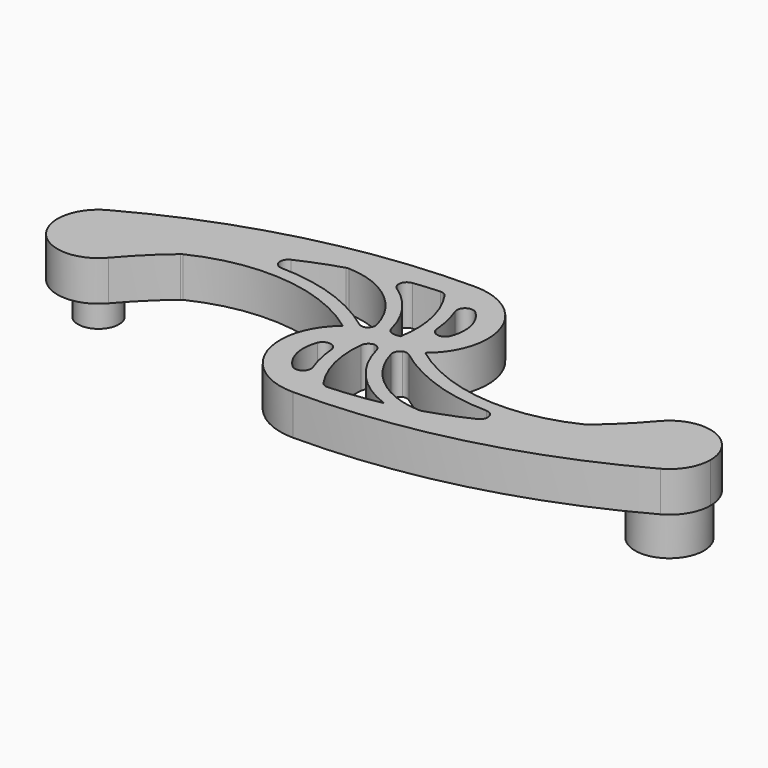
from build123d import *

# Parameters (mm, degrees)
F0_R            = 3.175
F0_R_2          = 5.334
F0_R_3          = 3.2385
F1_DEPTH        = 6.223
F2_DEPTH        = 5.08
F3_DEPTH        = 6.477
F4_DEPTH        = 6.223
F4_COPIES_COUNT = 2
F6_T1_DEPTH     = 6.223


# Not quite as in the source:
# - a fillet or chamfer that OpenCascade refuses, or shapes differently, is made with other operations: its cross-section is extruded or revolved along the edge and cut away or added
# - a pattern or mirror of a feature is missing from the dataset's text; its kind, count and spacing are read off the source's solid
# - a feature names something its author has since deleted; it is built from what else it names


with BuildPart() as f1:
    # F0 (on Top) → F1 (new body)
    with BuildSketch(Plane.XY):
        with BuildLine():
            ThreePointArc((-39.383509083, -4.1130659459), (-38.2614038875, -2.1911061906), (-37.8714, 0))
            ThreePointArc((-37.8714, 0), (-40.9830590014, 5.4622017152), (-47.268454355, 5.5711722068))
            ThreePointArc((-47.268454355, 5.5711722068), (-49.1456147646, -4.0093152723), (-39.383509083, -4.1130659459))
        make_face()
        with Locations((-44.2214, 0)):
            Circle(F0_R, mode=Mode.SUBTRACT)
        with BuildLine():
            ThreePointArc((-47.268454355, 5.5711722068), (-40.9830590014, 5.4622017152), (-37.8714, 0))
            ThreePointArc((-37.8714, 0), (-38.2614038875, -2.1911061906), (-39.383509083, -4.1130659459))
            ThreePointArc((-39.383509083, -4.1130659459), (-36.3513275231, -0.8434709111), (-33.0486454257, 2.1526378433))
            ThreePointArc((-33.0486454257, 2.1526378433), (-30.2955035901, 4.2889551927), (-27.404684246, 6.2349267505))
            ThreePointArc((-27.404684246, 6.2349267505), (-21.4521533969, 9.4356034701), (-15.1329284561, 11.8323410696))
            ThreePointArc((-15.1329284561, 11.8323410696), (-12.7951555369, 12.4884323965), (-10.4291525282, 13.0340218145))
            ThreePointArc((-10.4291525282, 13.0340218145), (-6.1458763765, 13.7303526951), (-1.8192889749, 14.0649759791))
            ThreePointArc((-1.8192889749, 14.0649759791), (-0.9097854022, 14.0889933747), (0, 14.097))
            ThreePointArc((0, 14.097), (0.3233426245, 14.0885072181), (0.6457935928, 14.0630522923))
            ThreePointArc((0.6457935928, 14.0630522923), (6.0043722729, 9.3111643906), (3.2449318821, 2.7020575802))
            ThreePointArc((3.2449318821, 2.7020575802), (2.1979242887, 2.1834953883), (1.0718312901, 1.8719729878))
            ThreePointArc((1.0718312901, 1.8719729878), (0.5379714762, 1.801538222), (0, 1.778))
            ThreePointArc((0, 1.778), (-0.4196313816, 1.7689334209), (-0.8384795567, 1.7417506054))
            ThreePointArc((-0.8384795567, 1.7417506054), (-1.8462351917, 1.6009671655), (-2.8337391369, 1.3555545438))
            ThreePointArc((-2.8337391369, 1.3555545438), (-3.5575469364, 1.1032300615), (-4.2592096932, 0.7946287805))
            ThreePointArc((-4.2592096932, 0.7946287805), (-5.2044321405, 0.2664518736), (-6.0850110833, -0.3636251419))
            ThreePointArc((-6.0850110833, -0.3636251419), (-9.1644672904, -11.1629425329), (0, -17.653))
            ThreePointArc((0, -17.653), (24.3940430225, -14.5847588813), (47.268454355, -5.5711722068))
            ThreePointArc((47.268454355, -5.5711722068), (39.2971852354, -4.0093152723), (39.383509083, 4.1130659459))
            ThreePointArc((39.383509083, 4.1130659459), (21.6948570487, -9.3241427599), (0, -14.097))
            ThreePointArc((0, -14.097), (-6.1595, -7.9375), (0, -1.778))
            ThreePointArc((0, -1.778), (9.7155, 7.9375), (0, 17.653))
            ThreePointArc((0, 17.653), (-24.3940430225, 14.5847588813), (-47.268454355, 5.5711722068))
        make_face()
        with BuildLine():
            ThreePointArc((50.5714, 0), (46.4125061906, 5.9599961125), (39.383509083, 4.1130659459))
            ThreePointArc((39.383509083, 4.1130659459), (39.2971852354, -4.0093152723), (47.268454355, -5.5711722068))
            ThreePointArc((47.268454355, -5.5711722068), (49.6836017152, -3.2383409986), (50.5714, 0))
        make_face()
        with Locations((44.2214, 0)):
            Circle(F0_R_2, mode=Mode.SUBTRACT)
        with Locations((-44.2214, 0)):
            Circle(F0_R)
        with Locations((44.2214, 0)):
            Circle(F0_R_2)
        with Locations((44.2214, 0)):
            Circle(F0_R_3, mode=Mode.SUBTRACT)
        with Locations((44.2214, 0)):
            Circle(F0_R_3)
    extrude(amount=F1_DEPTH)

    # F0 (on Top) → F2 (join)
    with BuildSketch(Plane.XY):
        with Locations((-44.2214, 0)):
            Circle(F0_R)
    extrude(amount=-F2_DEPTH)

    # F0 (on Top) → F3 (join)
    with BuildSketch(Plane.XY):
        with Locations((44.2214, 0)):
            Circle(F0_R_2)
        with Locations((44.2214, 0)):
            Circle(F0_R_3, mode=Mode.SUBTRACT)
    extrude(amount=-F3_DEPTH)

    # F0 (on Top) → F4 (join, through all)
    with BuildSketch(Plane.XY):
        with BuildLine():
            ThreePointArc((0, 14.097), (-0.9097854022, 14.0889933747), (-1.8192889749, 14.0649759791))
            ThreePointArc((-1.8192889749, 14.0649759791), (0.8983347122, 8.270097367), (1.0718312901, 1.8719729878))
            ThreePointArc((1.0718312901, 1.8719729878), (2.1979242887, 2.1834953883), (3.2449318821, 2.7020575802))
            ThreePointArc((3.2449318821, 2.7020575802), (2.9072627287, 8.6026158694), (0.6457935928, 14.0630522923))
            ThreePointArc((0.6457935928, 14.0630522923), (0.3233426245, 14.0885072181), (0, 14.097))
        make_face()
        with BuildLine():
            ThreePointArc((-27.404684246, 6.2349267505), (-30.2955035901, 4.2889551927), (-33.0486454257, 2.1526378433))
            ThreePointArc((-33.0486454257, 2.1526378433), (-19.2120899123, 4.6957922264), (-6.0850110833, -0.3636251419))
            ThreePointArc((-6.0850110833, -0.3636251419), (-5.2044321405, 0.2664518736), (-4.2592096932, 0.7946287805))
            ThreePointArc((-4.2592096932, 0.7946287805), (-15.2246797453, 6.09836568), (-27.404684246, 6.2349267505))
        make_face()
        with BuildLine():
            ThreePointArc((-10.4291525282, 13.0340218145), (-12.7951555369, 12.4884323965), (-15.1329284561, 11.8323410696))
            ThreePointArc((-15.1329284561, 11.8323410696), (-7.0940173553, 8.8119046713), (-2.8337391369, 1.3555545438))
            ThreePointArc((-2.8337391369, 1.3555545438), (-1.8462351917, 1.6009671655), (-0.8384795567, 1.7417506054))
            ThreePointArc((-0.8384795567, 1.7417506054), (-4.1057324321, 8.6857075171), (-10.4291525282, 13.0340218145))
        make_face()
    f4 = extrude(amount=F4_DEPTH)

    # F4_copies: F4 ×2 about axis
    f4_copies_axis = Axis((0, 0, 0), (0, 0, 1))
    for i in range(1, F4_COPIES_COUNT):
        add(f4.rotate(f4_copies_axis, i * 360 / F4_COPIES_COUNT))

    # F6: fillet of radius 1.27 on 20 edges, made by hand

    # F6_s2 → F6_t1 (join)
    with BuildSketch(Plane.XY):
        with BuildLine():
            ThreePointArc((5.7467371781, 5.7206436546), (4.3797028383, 4.920856325), (3.2959395861, 6.0758021557))
            ThreePointArc((3.2959395861, 6.0758021557), (3.351011683, 4.3877116388), (3.2449318821, 2.7020575802))
            ThreePointArc((3.2449318821, 2.7020575802), (4.7424143212, 4.006985192), (5.7467371781, 5.7206436546))
        make_face()
        with BuildLine():
            ThreePointArc((0.2264659862, 1.7821646389), (-0.5831545016, 2.0360014635), (-1.052242498, 2.7430197937))
            Line((-1.052242498, 2.7430197937), (-1.1754439447, 2.712191178))
            ThreePointArc((-1.1754439447, 2.712191178), (-1.0608351081, 2.2177324095), (-0.9635293288, 1.719579577))
            Line((-0.9635293288, 1.719579577), (-0.8275190397, 1.6152244537))
            ThreePointArc((-0.8275190397, 1.6152244537), (0, 1.651), (0.231135388, 1.6552505078))
            Line((0.231135388, 1.6552505078), (0.2264659862, 1.7821646389))
        make_face()
        with BuildLine():
            ThreePointArc((-6.5568541784, 13.6794711792), (-7.6316183523, 12.7122452972), (-7.104466753, 11.3658593468))
            ThreePointArc((-7.104466753, 11.3658593468), (-8.7137881282, 12.3056136619), (-10.4291525282, 13.0340218145))
            ThreePointArc((-10.4291525282, 13.0340218145), (-8.499132731, 13.3935189853), (-6.5568541784, 13.6794711792))
        make_face()
        with BuildLine():
            ThreePointArc((-21.8345577233, 9.259295464), (-22.5395513885, 7.8402717016), (-21.3121358485, 6.8382259948))
            ThreePointArc((-21.3121358485, 6.8382259948), (-24.3749772665, 6.7038840327), (-27.404684246, 6.2349267505))
            ThreePointArc((-27.404684246, 6.2349267505), (-24.6660178983, 7.832562553), (-21.8345577233, 9.259295464))
        make_face()
        with BuildLine():
            ThreePointArc((-3.0884774271, 2.4987897599), (-3.1708710573, 1.612134008), (-3.8152433992, 0.9975354255))
            ThreePointArc((-3.8152433992, 0.9975354255), (-3.3293072273, 1.1897478676), (-2.8337391369, 1.3555545438))
            ThreePointArc((-2.8337391369, 1.3555545438), (-2.9478756761, 1.9301206714), (-3.0884774271, 2.4987897599))
        make_face()
        with BuildLine():
            ThreePointArc((-3.6099534742, 1.0824321596), (-4.2483858683, 1.0024755302), (-4.844071044, 1.2456794691))
            ThreePointArc((-4.844071044, 1.2456794691), (-4.5501505396, 1.0220859329), (-4.2592096932, 0.7946287805))
            ThreePointArc((-4.2592096932, 0.7946287805), (-3.9372122034, 0.9444648904), (-3.6099534742, 1.0824321596))
        make_face()
        with BuildLine():
            ThreePointArc((-33.1684913048, 2.052686828), (-33.0427467511, 2.1453555086), (-32.9065771816, 2.2218867145))
            ThreePointArc((-32.9065771816, 2.2218867145), (-32.9776640835, 2.1873705598), (-33.0486454257, 2.1526378433))
            ThreePointArc((-33.0486454257, 2.1526378433), (-33.1086060828, 2.1027075608), (-33.1684913048, 2.052686828))
        make_face()
        with BuildLine():
            ThreePointArc((-15.3316650678, 11.7710586074), (-15.1263951869, 11.8165832907), (-14.9164273754, 11.8276168263))
            ThreePointArc((-14.9164273754, 11.8276168263), (-15.024667811, 11.8304420223), (-15.1329284561, 11.8323410696))
            ThreePointArc((-15.1329284561, 11.8323410696), (-15.2323275808, 11.8017997828), (-15.3316650678, 11.7710586074))
        make_face()
        with BuildLine():
            ThreePointArc((-2.5135222626, 14.0358550855), (-1.8858921716, 13.9043192732), (-1.4025369095, 13.4829063028))
            ThreePointArc((-1.4025369095, 13.4829063028), (-1.6075880681, 13.7763216947), (-1.8192889749, 14.0649759791))
            ThreePointArc((-1.8192889749, 14.0649759791), (-2.1664545487, 14.0515820074), (-2.5135222626, 14.0358550855))
        make_face()
        with BuildLine():
            ThreePointArc((33.1684913048, -2.052686828), (33.0427467511, -2.1453555086), (32.9065771816, -2.2218867145))
            ThreePointArc((32.9065771816, -2.2218867145), (32.9776640835, -2.1873705598), (33.0486454257, -2.1526378433))
            ThreePointArc((33.0486454257, -2.1526378433), (33.1086060828, -2.1027075608), (33.1684913048, -2.052686828))
        make_face()
        with BuildLine():
            ThreePointArc((15.3316650678, -11.7710586074), (15.1263951869, -11.8165832907), (14.9164273754, -11.8276168263))
            ThreePointArc((14.9164273754, -11.8276168263), (15.024667811, -11.8304420223), (15.1329284561, -11.8323410696))
            ThreePointArc((15.1329284561, -11.8323410696), (15.2323275808, -11.8017997828), (15.3316650678, -11.7710586074))
        make_face()
        with BuildLine():
            ThreePointArc((21.8345577233, -9.259295464), (22.5395513885, -7.8402717016), (21.3121358485, -6.8382259948))
            ThreePointArc((21.3121358485, -6.8382259948), (24.3749772665, -6.7038840327), (27.404684246, -6.2349267505))
            ThreePointArc((27.404684246, -6.2349267505), (24.6660178983, -7.832562553), (21.8345577233, -9.259295464))
        make_face()
        with BuildLine():
            ThreePointArc((2.5135222626, -14.0358550855), (1.8858921716, -13.9043192732), (1.4025369095, -13.4829063028))
            ThreePointArc((1.4025369095, -13.4829063028), (1.6075880681, -13.7763216947), (1.8192889749, -14.0649759791))
            ThreePointArc((1.8192889749, -14.0649759791), (2.1664545487, -14.0515820074), (2.5135222626, -14.0358550855))
        make_face()
        with BuildLine():
            ThreePointArc((-5.7467371781, -5.7206436546), (-4.3797028383, -4.920856325), (-3.2959395861, -6.0758021557))
            ThreePointArc((-3.2959395861, -6.0758021557), (-3.351011683, -4.3877116388), (-3.2449318821, -2.7020575802))
            ThreePointArc((-3.2449318821, -2.7020575802), (-4.7424143212, -4.006985192), (-5.7467371781, -5.7206436546))
        make_face()
        with BuildLine():
            ThreePointArc((-4.2112141477, -12.4325100836), (-2.6324155303, -12.5583575491), (-2.1586241483, -11.0470784931))
            ThreePointArc((-2.1586241483, -11.0470784931), (-1.4742400944, -12.5911966868), (-0.6457935928, -14.0630522923))
            ThreePointArc((-0.6457935928, -14.0630522923), (-2.561698269, -13.539030347), (-4.2112141477, -12.4325100836))
        make_face()
        with BuildLine():
            ThreePointArc((0.0344635389, -1.777938874), (-0.8091247214, -2.1026067288), (-1.2230924584, -2.90614956))
            Line((-1.2230924584, -2.90614956), (-1.3492985619, -2.8919714276))
            ThreePointArc((-1.3492985619, -2.8919714276), (-1.2817508345, -2.3694198456), (-1.1968113014, -1.8494120311))
            Line((-1.1968113014, -1.8494120311), (-1.0939309043, -1.7469105752))
            ThreePointArc((-1.0939309043, -1.7469105752), (0, -1.651), (0.0340130351, -1.650939673))
            Line((0.0340130351, -1.650939673), (0.0344635389, -1.777938874))
        make_face()
        with BuildLine():
            ThreePointArc((-0.2264659862, -1.7821646389), (0.5831545016, -2.0360014635), (1.052242498, -2.7430197937))
            Line((1.052242498, -2.7430197937), (1.1754439447, -2.712191178))
            ThreePointArc((1.1754439447, -2.712191178), (1.0608351081, -2.2177324095), (0.9635293288, -1.719579577))
            Line((0.9635293288, -1.719579577), (0.8275190397, -1.6152244537))
            ThreePointArc((0.8275190397, -1.6152244537), (0, -1.651), (-0.231135388, -1.6552505078))
            Line((-0.231135388, -1.6552505078), (-0.2264659862, -1.7821646389))
        make_face()
        with BuildLine():
            ThreePointArc((3.6099534742, -1.0824321596), (4.2483858683, -1.0024755302), (4.844071044, -1.2456794691))
            ThreePointArc((4.844071044, -1.2456794691), (4.5501505396, -1.0220859329), (4.2592096932, -0.7946287805))
            ThreePointArc((4.2592096932, -0.7946287805), (3.9372122034, -0.9444648904), (3.6099534742, -1.0824321596))
        make_face()
        with BuildLine():
            ThreePointArc((3.8152433992, -0.9975354255), (3.1708710573, -1.612134008), (3.0884774271, -2.4987897599))
            ThreePointArc((3.0884774271, -2.4987897599), (2.9478756761, -1.9301206714), (2.8337391369, -1.3555545438))
            ThreePointArc((2.8337391369, -1.3555545438), (3.3293072273, -1.1897478676), (3.8152433992, -0.9975354255))
        make_face()
        with BuildLine():
            ThreePointArc((4.2112141477, 12.4325100836), (2.6324155303, 12.5583575491), (2.1586241483, 11.0470784931))
            ThreePointArc((2.1586241483, 11.0470784931), (1.4742400944, 12.5911966868), (0.6457935928, 14.0630522923))
            ThreePointArc((0.6457935928, 14.0630522923), (2.561698269, 13.539030347), (4.2112141477, 12.4325100836))
        make_face()
    extrude(amount=F6_T1_DEPTH)


solid = f1.part
